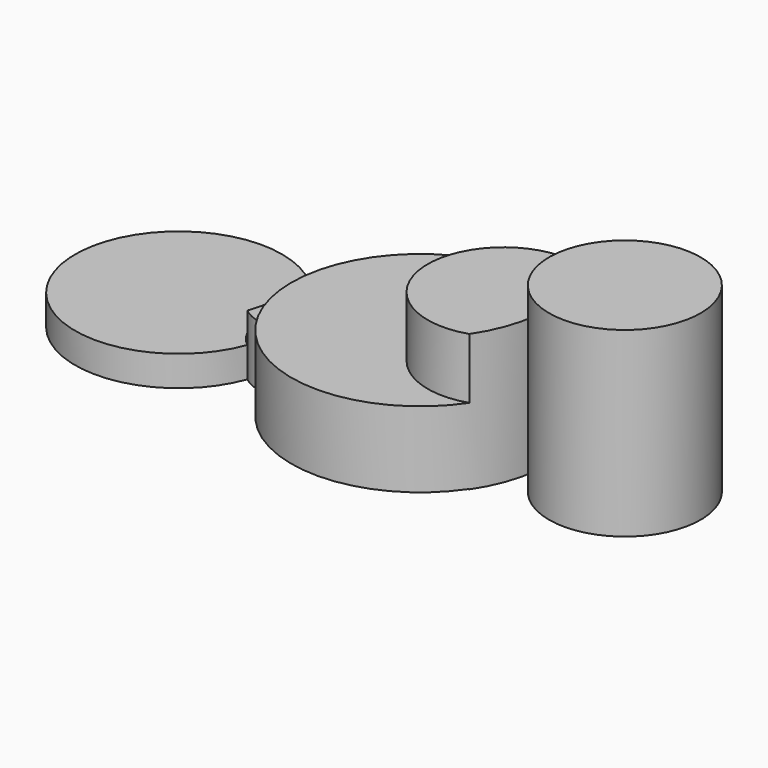
from build123d import *

# Parameters (mm, degrees)
F1_DEPTH      = 12000
F2_DEPTH      = 9000
F2_DEPTH_BACK = 25
F3_DEPTH      = 5000
F4_DEPTH      = 4000
F5_DEPTH      = 2000


# Not quite as in the source:
# - a feature names something its author has since deleted; it is built from what else it names


with BuildPart() as f1:
    # F0 (on Top) → F1 (new body)
    with BuildSketch(Plane.XY):
        with BuildLine():
            ThreePointArc((-4000, -3000), (1581.1388300842, -4743.4164902526), (5000, 0))
            ThreePointArc((5000, 0), (1581.1388300842, 4743.4164902526), (-4000, 3000))
            ThreePointArc((-4000, 3000), (-3256.5835097474, 1581.1388300842), (-3000, 0))
            ThreePointArc((-3000, 0), (-3256.5835097474, -1581.1388300842), (-4000, -3000))
        make_face()
        with BuildLine():
            ThreePointArc((-3000, 0), (-3256.5835097474, 1581.1388300842), (-4000, 3000))
            ThreePointArc((-4000, 3000), (-4743.4164902526, 1581.1388300842), (-5000, 0))
            ThreePointArc((-5000, 0), (-4743.4164902526, -1581.1388300842), (-4000, -3000))
            ThreePointArc((-4000, -3000), (-3256.5835097474, -1581.1388300842), (-3000, 0))
        make_face()
    extrude(amount=F1_DEPTH)

    # F0 (on Top) → F2 (join, two sides)
    with BuildSketch(Plane.XY) as f2_sk:
        with BuildLine():
            ThreePointArc((-5000, 0), (-4743.4164902526, 1581.1388300842), (-4000, 3000))
            ThreePointArc((-4000, 3000), (-5091.7074828837, 4067.1654299875), (-6454.5454545455, 4755.1624838626))
            ThreePointArc((-6454.5454545455, 4755.1624838626), (-5371.7663777312, 2486.3262420323), (-5000, 0))
        make_face()
        with BuildLine():
            ThreePointArc((-6454.5454545455, -4755.1624838626), (-5371.7663777312, -2486.3262420323), (-5000, 0))
            ThreePointArc((-5000, 0), (-5371.7663777312, 2486.3262420323), (-6454.5454545455, 4755.1624838626))
            ThreePointArc((-6454.5454545455, 4755.1624838626), (-13000, 0), (-6454.5454545456, -4755.1624838626))
        make_face()
    extrude(amount=F2_DEPTH)
    extrude(f2_sk.sketch, amount=-F2_DEPTH_BACK)

    # F0 (on Top) → F3 (join)
    with BuildSketch(Plane.XY):
        with BuildLine():
            ThreePointArc((-18161.2319946289, 0), (-19147.7686227754, 2223.9526186959), (-21458.5421614318, 2985.2314256546))
            ThreePointArc((-21458.5421614317, 2985.2314256544), (-22000, 0), (-21458.5421614317, -2985.2314256544))
            ThreePointArc((-21458.5421614318, -2985.2314256546), (-19147.7686227754, -2223.9526186959), (-18161.2319946289, 0))
        make_face()
        with BuildLine():
            ThreePointArc((-6454.5454545456, -4755.1624838626), (-13000, 0), (-6454.5454545455, 4755.1624838626))
            ThreePointArc((-6454.5454545455, 4755.1624838626), (-14495.7892529623, 8441.4692893882), (-21458.5421614317, 2985.2314256544))
            ThreePointArc((-21458.5421614318, 2985.2314256546), (-19147.7686227754, 2223.9526186959), (-18161.2319946289, 0))
            ThreePointArc((-18161.2319946289, 0), (-19147.7686227754, -2223.9526186959), (-21458.5421614318, -2985.2314256546))
            ThreePointArc((-21458.5421614317, -2985.2314256544), (-14495.7892529623, -8441.4692893882), (-6454.5454545455, -4755.1624838626))
        make_face()
    extrude(amount=F3_DEPTH)

    # F0 (on Top) → F4 (join)
    with BuildSketch(Plane.XY):
        with BuildLine():
            ThreePointArc((-21458.5421614317, -2985.2314256544), (-22000, 0), (-21458.5421614317, 2985.2314256544))
            ThreePointArc((-21458.5421614318, 2985.2314256546), (-22283.7629869561, 2782.0719205773), (-23018.8990545433, 2355.6470649291))
            ThreePointArc((-23018.8990545434, 2355.6470649291), (-22705.4436981203, 1196.3128526148), (-22599.8708086972, 0))
            ThreePointArc((-22599.8708086972, 0), (-22705.4436981203, -1196.3128526148), (-23018.8990545434, -2355.6470649291))
            ThreePointArc((-23018.8990545433, -2355.6470649291), (-22283.7629869561, -2782.0719205773), (-21458.5421614318, -2985.2314256546))
        make_face()
    extrude(amount=F4_DEPTH)

    # F0 (on Top) → F5 (join)
    with BuildSketch(Plane.XY):
        with BuildLine():
            ThreePointArc((-23018.8990545433, -2355.6470649291), (-24161.2319946289, 0), (-23018.8990545433, 2355.6470649291))
            ThreePointArc((-23018.8990545434, 2355.6470649291), (-36261.6175335879, 0), (-23018.8990545434, -2355.6470649291))
        make_face()
    extrude(amount=F5_DEPTH)


solid = f1.part
